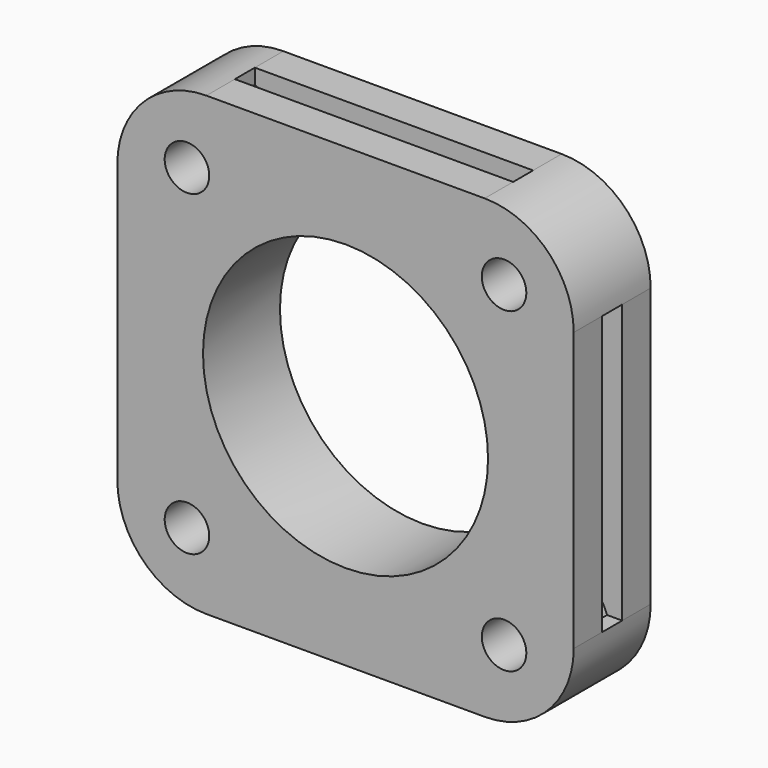
from build123d import *

# Parameters (mm, degrees)
F0_R     = 1.5875
F0_R_2   = 10.16
F1_DEPTH = 6.858
F2_T     = 2.54


# Not quite as in the source:
# - a shell that OpenCascade refuses in one call is made with other operations: the cavity is built on its own and cut out


with BuildPart() as f1:
    # F0 (on Front) → F1 (new body)
    with BuildSketch(Plane.XZ):
        with BuildLine():
            Line((9.9187, 16.2687), (-9.9187, 16.2687))
            ThreePointArc((-9.9187, 16.2687), (-14.4088280605, 14.4088280605), (-16.2687, 9.9187))
            Line((-16.2687, 9.9187), (-16.2687, -9.9187))
            ThreePointArc((-16.2687, -9.9187), (-14.4088280605, -14.4088280605), (-9.9187, -16.2687))
            Line((-9.9187, -16.2687), (9.9187, -16.2687))
            ThreePointArc((9.9187, -16.2687), (14.4088280605, -14.4088280605), (16.2687, -9.9187))
            Line((16.2687, -9.9187), (16.2687, 9.9187))
            ThreePointArc((16.2687, 9.9187), (14.4088280605, 14.4088280605), (9.9187, 16.2687))
        make_face()
        with Locations((-11.303, -11.303)):
            Circle(F0_R, mode=Mode.SUBTRACT)
        with Locations((11.303, -11.303)):
            Circle(F0_R, mode=Mode.SUBTRACT)
        with Locations((-11.303, 11.303)):
            Circle(F0_R, mode=Mode.SUBTRACT)
        Circle(F0_R_2, mode=Mode.SUBTRACT)
        with Locations((11.303, 11.303)):
            Circle(F0_R, mode=Mode.SUBTRACT)
    extrude(amount=F1_DEPTH)

    # F2: shell of thickness 2.54, made by hand


with BuildPart() as f2_core1:
    # F2_t2: copy of F1
    add(f1.part)

    # the walls: a layer under each face that stays
    f2_faces = [f2_core1.faces().sort_by_distance(p)[0] for p in [
        (-14.4088280605, -3.429, 14.4088280605),
        (-14.4088280605, -3.429, -14.4088280605),
        (14.4088280605, -3.429, -14.4088280605),
        (14.4088280605, -3.429, 14.4088280605),
        (-12.8905, -3.429, -11.303),
        (9.7155, -3.429, -11.303),
        (-12.8905, -3.429, 11.303),
        (-10.16, -3.429, 0),
        (9.7155, -3.429, 11.303),
        (-10.8458, 0, 0),
        (-10.8458, -6.858, 0),
    ]]
    thicken(f2_faces, amount=-F2_T, mode=Mode.SUBTRACT)


with BuildPart() as f1_1:
    add(f1.part)

    # what is left inside the walls is the cavity
    f2_cavity = [f2_core1.part.solids().sort_by_distance(p)[0] for p in [
        (-4.95935, -4.2926, 14.316209),
        (13.339963, -4.2926, -3.306233),
        (-13.339963, -4.2926, -3.306233),
        (0, -2.5654, -14.316209),
    ]]
    add(f2_cavity, mode=Mode.SUBTRACT)


solid = f1_1.part
